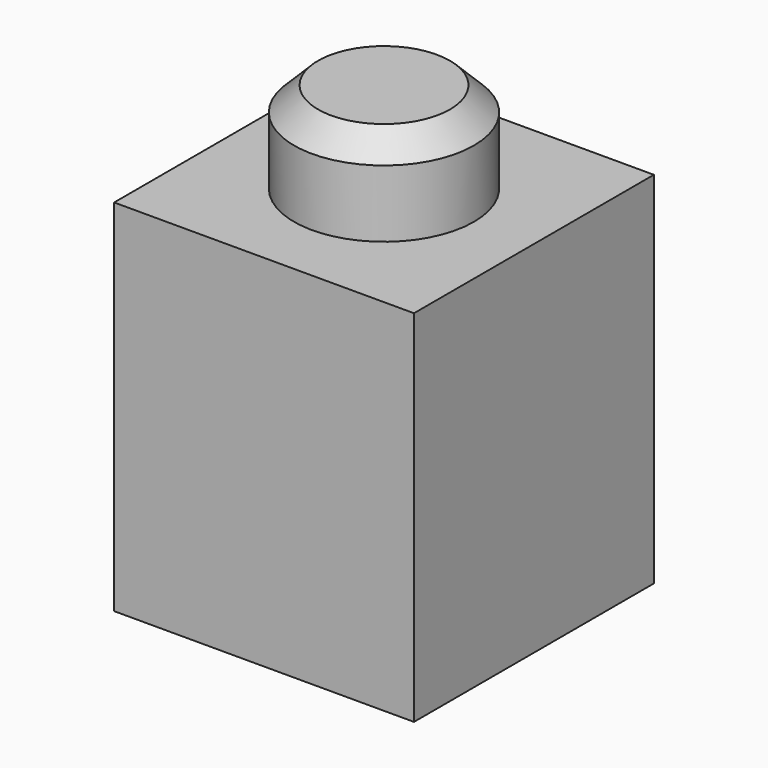
from build123d import *

# Parameters (mm, degrees)
F0_W     = 15.875
F0_H     = 19.05
F1_DEPTH = 7.9375
F2_R     = 4.7625
F3_DEPTH = 4.826
F4_SIZE  = 1.27
F5_T     = -1.5875


with BuildPart() as f1:
    # F0 (on Front) → F1 (new body, symmetric)
    with BuildSketch(Plane.XZ):
        Rectangle(F0_W, F0_H)
    extrude(amount=F1_DEPTH, both=True)

    # F2 (on face) → F3 (join)
    with BuildSketch(Plane.XY.offset(9.525)):
        Circle(F2_R)
    extrude(amount=F3_DEPTH)

    # F4
    f4_edges = [f1.edges().sort_by_distance(p)[0] for p in [
        (-4.7625, 0, 14.351),
    ]]
    chamfer(f4_edges, length=F4_SIZE)

    # F5
    f5_openings = [f1.faces().sort_by_distance(p)[0] for p in [
        (0, 0, -9.525),
    ]]
    offset(amount=F5_T, openings=f5_openings, kind=Kind.INTERSECTION)


solid = f1.part
